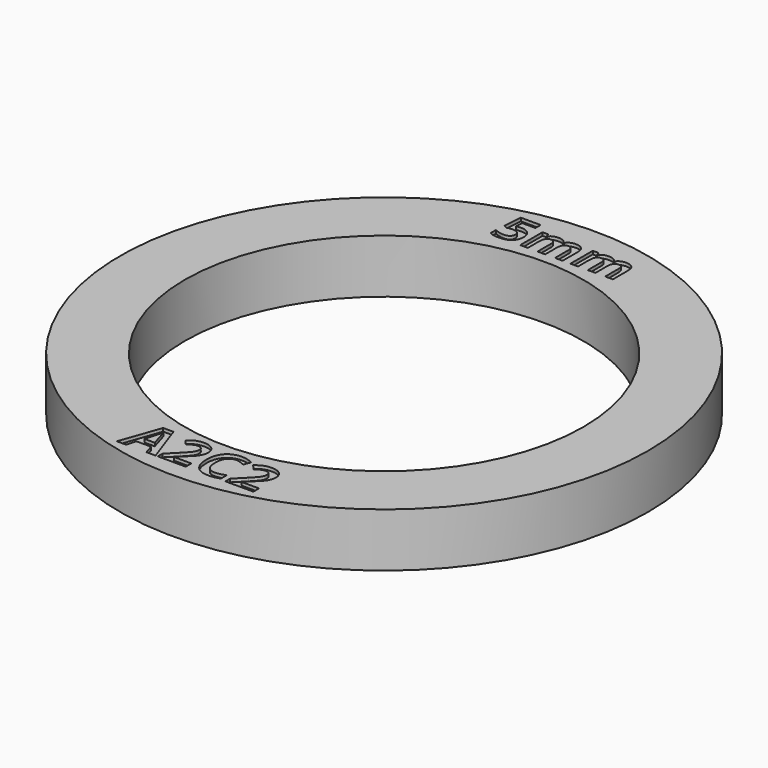
from build123d import *

# Parameters (mm, degrees)
F0_R           = 24.5
F0_R_2         = 18.5
F0_TEXT_SIZE   = 5.1974965673
F0_TEXT_SIZE_2 = 4.7515974277
F1_DEPTH       = 5
F2_DEPTH       = 0.3


# Not quite as in the source:
# - Text() gives the source's letters only with a copy of the font that has no kerning and outlines rounded to 1/6400 em; it was checked with that copy


with BuildPart() as f1:
    # F0 (on Top) → F1 (new body)
    with BuildSketch(Plane.XY):
        Circle(F0_R)
        Polygon((-2.9154707307, -22.8730905801), (-3.7633123583, -22.8730905801), (-4.0321203839, -21.9895161637), (-5.3850937091, -21.9895161637), (-5.6539017347, -22.8730905801), (-6.5017433622, -22.8730905801), (-5.1918118055, -19.1471352284), (-4.2302749405, -19.1471352284), align=None, mode=Mode.SUBTRACT)
        with BuildLine():
            Line((-0.1136952374, -22.2128460943), (-0.1136952374, -22.8730905801))
            Line((-0.1136952374, -22.8730905801), (-2.707570868, -22.8730905801))
            Line((-2.707570868, -22.8730905801), (-2.707570868, -22.3273534405))
            Line((-2.707570868, -22.3273534405), (-1.7760820301, -21.3861192965))
            add(Edge.make_bspline(
                [(-1.7760820301, -21.3861192965), (-1.3619065224, -20.9621984828), (-1.2352175436, -20.7985585518)],
                knots=[0, 0, 0, 1, 1, 1], degree=2))
            add(Edge.make_bspline(
                [(-1.2352175436, -20.7985585518), (-1.1085285648, -20.6349186208), (-1.0524930549, -20.4952359005)],
                knots=[0, 0, 0, 1, 1, 1], degree=2))
            add(Edge.make_bspline(
                [(-1.0524930549, -20.4952359005), (-0.996457545, -20.3555531803), (-0.996457545, -20.206125154)],
                knots=[0, 0, 0, 1, 1, 1], degree=2))
            add(Edge.make_bspline(
                [(-0.996457545, -20.206125154), (-0.996457545, -19.9827952234), (-1.1198980885, -19.8735665846)],
                knots=[0, 0, 0, 1, 1, 1], degree=2))
            add(Edge.make_bspline(
                [(-1.1198980885, -19.8735665846), (-1.243338632, -19.7643379458), (-1.4488021681, -19.7643379458)],
                knots=[0, 0, 0, 1, 1, 1], degree=2))
            add(Edge.make_bspline(
                [(-1.4488021681, -19.7643379458), (-1.6640110104, -19.7643379458), (-1.86703822, -19.8634152241)],
                knots=[0, 0, 0, 1, 1, 1], degree=2))
            add(Edge.make_bspline(
                [(-1.86703822, -19.8634152241), (-2.0700654297, -19.9624925024), (-2.2909590338, -20.1452169911)],
                knots=[0, 0, 0, 1, 1, 1], degree=2))
            Line((-2.2909590338, -20.1452169911), (-2.7173161741, -19.6400852935))
            add(Edge.make_bspline(
                [(-2.7173161741, -19.6400852935), (-2.4436354955, -19.4061979479), (-2.2633473333, -19.3099630505)],
                knots=[0, 0, 0, 1, 1, 1], degree=2))
            add(Edge.make_bspline(
                [(-2.2633473333, -19.3099630505), (-2.0830591711, -19.2137281532), (-1.869880601, -19.1617531875)],
                knots=[0, 0, 0, 1, 1, 1], degree=2))
            add(Edge.make_bspline(
                [(-1.869880601, -19.1617531875), (-1.6567020308, -19.1097782218), (-1.3927666583, -19.1097782218)],
                knots=[0, 0, 0, 1, 1, 1], degree=2))
            add(Edge.make_bspline(
                [(-1.3927666583, -19.1097782218), (-1.0451840753, -19.1097782218), (-0.7788123763, -19.2364672006)],
                knots=[0, 0, 0, 1, 1, 1], degree=2))
            add(Edge.make_bspline(
                [(-0.7788123763, -19.2364672006), (-0.5124406772, -19.3631561795), (-0.365042923, -19.5917648176)],
                knots=[0, 0, 0, 1, 1, 1], degree=2))
            add(Edge.make_bspline(
                [(-0.365042923, -19.5917648176), (-0.2176451688, -19.8203734556), (-0.2176451688, -20.1143568552)],
                knots=[0, 0, 0, 1, 1, 1], degree=2))
            add(Edge.make_bspline(
                [(-0.2176451688, -20.1143568552), (-0.2176451688, -20.3709832482), (-0.3077892498, -20.5955313421)],
                knots=[0, 0, 0, 1, 1, 1], degree=2))
            add(Edge.make_bspline(
                [(-0.3077892498, -20.5955313421), (-0.3979333309, -20.820079436), (-0.5871546903, -21.0559970536)],
                knots=[0, 0, 0, 1, 1, 1], degree=2))
            add(Edge.make_bspline(
                [(-0.5871546903, -21.0559970536), (-0.7763760497, -21.2919146713), (-1.253083938, -21.7288292265)],
                knots=[0, 0, 0, 1, 1, 1], degree=2))
            Line((-1.253083938, -21.7288292265), (-1.7306039352, -22.1779254142))
            Line((-1.7306039352, -22.1779254142), (-1.7306039352, -22.2128460943))
            Line((-1.7306039352, -22.2128460943), (-0.1136952374, -22.2128460943))
        make_face(mode=Mode.SUBTRACT)
        Circle(F0_R_2, mode=Mode.SUBTRACT)
        with BuildLine():
            add(Edge.make_bspline(
                [(2.5077920937, -19.8378337957), (2.2974559045, -19.7643379458), (2.0944286949, -19.7643379458)],
                knots=[0, 0, 0, 1, 1, 1], degree=2))
            add(Edge.make_bspline(
                [(2.0944286949, -19.7643379458), (1.6502051601, -19.7643379458), (1.4065725085, -20.0981146785)],
                knots=[0, 0, 0, 1, 1, 1], degree=2))
            add(Edge.make_bspline(
                [(1.4065725085, -20.0981146785), (1.1629398569, -20.4318914111), (1.1629398569, -21.0279792987)],
                knots=[0, 0, 0, 1, 1, 1], degree=2))
            add(Edge.make_bspline(
                [(1.1629398569, -21.0279792987), (1.1629398569, -22.2688816042), (2.0944286949, -22.2688816042)],
                knots=[0, 0, 0, 1, 1, 1], degree=2))
            add(Edge.make_bspline(
                [(2.0944286949, -22.2688816042), (2.4850530463, -22.2688816042), (3.0405354919, -22.0739754829)],
                knots=[0, 0, 0, 1, 1, 1], degree=2))
            Line((3.0405354919, -22.0739754829), (3.0405354919, -22.7334078599))
            add(Edge.make_bspline(
                [(3.0405354919, -22.7334078599), (2.5841303246, -22.9242534369), (2.0205267906, -22.9242534369)],
                knots=[0, 0, 0, 1, 1, 1], degree=2))
            add(Edge.make_bspline(
                [(2.0205267906, -22.9242534369), (1.2108542784, -22.9242534369), (0.7820608116, -22.4329275896)],
                knots=[0, 0, 0, 1, 1, 1], degree=2))
            add(Edge.make_bspline(
                [(0.7820608116, -22.4329275896), (0.3532673448, -21.9416017422), (0.3532673448, -21.0231066457)],
                knots=[0, 0, 0, 1, 1, 1], degree=2))
            add(Edge.make_bspline(
                [(0.3532673448, -21.0231066457), (0.3532673448, -20.4440730437), (0.5640095884, -20.0087827062)],
                knots=[0, 0, 0, 1, 1, 1], degree=2))
            add(Edge.make_bspline(
                [(0.5640095884, -20.0087827062), (0.7747518321, -19.5734923687), (1.1694367277, -19.3416352953)],
                knots=[0, 0, 0, 1, 1, 1], degree=2))
            add(Edge.make_bspline(
                [(1.1694367277, -19.3416352953), (1.5641216232, -19.1097782218), (2.0944286949, -19.1097782218)],
                knots=[0, 0, 0, 1, 1, 1], degree=2))
            add(Edge.make_bspline(
                [(2.0944286949, -19.1097782218), (2.6344810726, -19.1097782218), (3.1802182121, -19.370465159)],
                knots=[0, 0, 0, 1, 1, 1], degree=2))
            Line((3.1802182121, -19.370465159), (2.9268402545, -20.0104069239))
            add(Edge.make_bspline(
                [(2.9268402545, -20.0104069239), (2.7181282829, -19.9113296456), (2.5077920937, -19.8378337957)],
                knots=[0, 0, 0, 1, 1, 1], degree=2))
        make_face(mode=Mode.SUBTRACT)
        with BuildLine():
            Line((6.1647181942, -22.2128460943), (6.1647181942, -22.8730905801))
            Line((6.1647181942, -22.8730905801), (3.5708425635, -22.8730905801))
            Line((3.5708425635, -22.8730905801), (3.5708425635, -22.3273534405))
            Line((3.5708425635, -22.3273534405), (4.5023314015, -21.3861192965))
            add(Edge.make_bspline(
                [(4.5023314015, -21.3861192965), (4.9165069092, -20.9621984828), (5.043195888, -20.7985585518)],
                knots=[0, 0, 0, 1, 1, 1], degree=2))
            add(Edge.make_bspline(
                [(5.043195888, -20.7985585518), (5.1698848668, -20.6349186208), (5.2259203767, -20.4952359005)],
                knots=[0, 0, 0, 1, 1, 1], degree=2))
            add(Edge.make_bspline(
                [(5.2259203767, -20.4952359005), (5.2819558866, -20.3555531803), (5.2819558866, -20.206125154)],
                knots=[0, 0, 0, 1, 1, 1], degree=2))
            add(Edge.make_bspline(
                [(5.2819558866, -20.206125154), (5.2819558866, -19.9827952234), (5.1585153431, -19.8735665846)],
                knots=[0, 0, 0, 1, 1, 1], degree=2))
            add(Edge.make_bspline(
                [(5.1585153431, -19.8735665846), (5.0350747996, -19.7643379458), (4.8296112634, -19.7643379458)],
                knots=[0, 0, 0, 1, 1, 1], degree=2))
            add(Edge.make_bspline(
                [(4.8296112634, -19.7643379458), (4.6144024212, -19.7643379458), (4.4113752115, -19.8634152241)],
                knots=[0, 0, 0, 1, 1, 1], degree=2))
            add(Edge.make_bspline(
                [(4.4113752115, -19.8634152241), (4.2083480019, -19.9624925024), (3.9874543978, -20.1452169911)],
                knots=[0, 0, 0, 1, 1, 1], degree=2))
            Line((3.9874543978, -20.1452169911), (3.5610972575, -19.6400852935))
            add(Edge.make_bspline(
                [(3.5610972575, -19.6400852935), (3.8347779361, -19.4061979479), (4.0150660983, -19.3099630505)],
                knots=[0, 0, 0, 1, 1, 1], degree=2))
            add(Edge.make_bspline(
                [(4.0150660983, -19.3099630505), (4.1953542604, -19.2137281532), (4.4085328306, -19.1617531875)],
                knots=[0, 0, 0, 1, 1, 1], degree=2))
            add(Edge.make_bspline(
                [(4.4085328306, -19.1617531875), (4.6217114007, -19.1097782218), (4.8856467733, -19.1097782218)],
                knots=[0, 0, 0, 1, 1, 1], degree=2))
            add(Edge.make_bspline(
                [(4.8856467733, -19.1097782218), (5.2332293562, -19.1097782218), (5.4996010553, -19.2364672006)],
                knots=[0, 0, 0, 1, 1, 1], degree=2))
            add(Edge.make_bspline(
                [(5.4996010553, -19.2364672006), (5.7659727544, -19.3631561795), (5.9133705086, -19.5917648176)],
                knots=[0, 0, 0, 1, 1, 1], degree=2))
            add(Edge.make_bspline(
                [(5.9133705086, -19.5917648176), (6.0607682628, -19.8203734556), (6.0607682628, -20.1143568552)],
                knots=[0, 0, 0, 1, 1, 1], degree=2))
            add(Edge.make_bspline(
                [(6.0607682628, -20.1143568552), (6.0607682628, -20.3709832482), (5.9706241817, -20.5955313421)],
                knots=[0, 0, 0, 1, 1, 1], degree=2))
            add(Edge.make_bspline(
                [(5.9706241817, -20.5955313421), (5.8804801006, -20.820079436), (5.6912587412, -21.0559970536)],
                knots=[0, 0, 0, 1, 1, 1], degree=2))
            add(Edge.make_bspline(
                [(5.6912587412, -21.0559970536), (5.5020373818, -21.2919146713), (5.0253294935, -21.7288292265)],
                knots=[0, 0, 0, 1, 1, 1], degree=2))
            Line((5.0253294935, -21.7288292265), (4.5478094964, -22.1779254142))
            Line((4.5478094964, -22.1779254142), (4.5478094964, -22.2128460943))
            Line((4.5478094964, -22.2128460943), (6.1647181942, -22.2128460943))
        make_face(mode=Mode.SUBTRACT)
        with BuildLine():
            add(Edge.make_bspline(
                [(-4.9238428344, 21.5662038617), (-4.7820373487, 21.598871094), (-4.5734125241, 21.598871094)],
                knots=[0, 0, 0, 1, 1, 1], degree=2))
            add(Edge.make_bspline(
                [(-4.5734125241, 21.598871094), (-4.0819191652, 21.598871094), (-3.7905126042, 21.3226844935)],
                knots=[0, 0, 0, 1, 1, 1], degree=2))
            add(Edge.make_bspline(
                [(-3.7905126042, 21.3226844935), (-3.4991060432, 21.046497893), (-3.4991060432, 20.5661410906)],
                knots=[0, 0, 0, 1, 1, 1], degree=2))
            add(Edge.make_bspline(
                [(-3.4991060432, 20.5661410906), (-3.4991060432, 19.9981767105), (-3.8495363535, 19.691550189)],
                knots=[0, 0, 0, 1, 1, 1], degree=2))
            add(Edge.make_bspline(
                [(-3.8495363535, 19.691550189), (-4.1999666638, 19.3849236675), (-4.8518264359, 19.3849236675)],
                knots=[0, 0, 0, 1, 1, 1], degree=2))
            add(Edge.make_bspline(
                [(-4.8518264359, 19.3849236675), (-5.4183059417, 19.3849236675), (-5.7657665036, 19.5683056308)],
                knots=[0, 0, 0, 1, 1, 1], degree=2))
            Line((-5.7657665036, 19.5683056308), (-5.7657665036, 20.1882406076))
            add(Edge.make_bspline(
                [(-5.7657665036, 20.1882406076), (-5.5831269775, 20.0909813478), (-5.3392363908, 20.0293590687)],
                knots=[0, 0, 0, 1, 1, 1], degree=2))
            add(Edge.make_bspline(
                [(-5.3392363908, 20.0293590687), (-5.0953458041, 19.9677367895), (-4.8778117343, 19.9677367895)],
                knots=[0, 0, 0, 1, 1, 1], degree=2))
            add(Edge.make_bspline(
                [(-4.8778117343, 19.9677367895), (-4.2207549025, 19.9677367895), (-4.2207549025, 20.5060036856)],
                knots=[0, 0, 0, 1, 1, 1], degree=2))
            add(Edge.make_bspline(
                [(-4.2207549025, 20.5060036856), (-4.2207549025, 21.0190277204), (-4.9008272844, 21.0190277204)],
                knots=[0, 0, 0, 1, 1, 1], degree=2))
            add(Edge.make_bspline(
                [(-4.9008272844, 21.0190277204), (-5.0233294056, 21.0190277204), (-5.1718168252, 20.9945272962)],
                knots=[0, 0, 0, 1, 1, 1], degree=2))
            add(Edge.make_bspline(
                [(-5.1718168252, 20.9945272962), (-5.3203042448, 20.9700268719), (-5.413108882, 20.9418142622)],
                knots=[0, 0, 0, 1, 1, 1], degree=2))
            Line((-5.413108882, 20.9418142622), (-5.6989471648, 21.0954987415))
            Line((-5.6989471648, 21.0954987415), (-5.5712479839, 22.8238923058))
            Line((-5.5712479839, 22.8238923058), (-3.7314888549, 22.8238923058))
            Line((-3.7314888549, 22.8238923058), (-3.7314888549, 22.2158363225))
            Line((-3.7314888549, 22.2158363225), (-4.9424037619, 22.2158363225))
            Line((-4.9424037619, 22.2158363225), (-5.0047684781, 21.5498702455))
            Line((-5.0047684781, 21.5498702455), (-4.9238428344, 21.5662038617))
        make_face(mode=Mode.SUBTRACT)
        with BuildLine():
            Line((-0.5924648043, 20.7331894376), (-0.5924648043, 19.4316972047))
            Line((-0.5924648043, 19.4316972047), (-1.3000073587, 19.4316972047))
            Line((-1.3000073587, 19.4316972047), (-1.3000073587, 20.9470113219))
            add(Edge.make_bspline(
                [(-1.3000073587, 20.9470113219), (-1.3000073587, 21.2276525449), (-1.3939256516, 21.3679731565)],
                knots=[0, 0, 0, 1, 1, 1], degree=2))
            add(Edge.make_bspline(
                [(-1.3939256516, 21.3679731565), (-1.4878439445, 21.508293768), (-1.6897868352, 21.508293768)],
                knots=[0, 0, 0, 1, 1, 1], degree=2))
            add(Edge.make_bspline(
                [(-1.6897868352, 21.508293768), (-1.9615188131, 21.508293768), (-2.0843921528, 21.3085781886)],
                knots=[0, 0, 0, 1, 1, 1], degree=2))
            add(Edge.make_bspline(
                [(-2.0843921528, 21.3085781886), (-2.2072654926, 21.1088626093), (-2.2072654926, 20.6522637939)],
                knots=[0, 0, 0, 1, 1, 1], degree=2))
            Line((-2.2072654926, 20.6522637939), (-2.2072654926, 19.4316972047))
            Line((-2.2072654926, 19.4316972047), (-2.914808047, 19.4316972047))
            Line((-2.914808047, 19.4316972047), (-2.914808047, 22.0257724254))
            Line((-2.914808047, 22.0257724254), (-2.3743138396, 22.0257724254))
            Line((-2.3743138396, 22.0257724254), (-2.2792818911, 21.6939030425))
            Line((-2.2792818911, 21.6939030425), (-2.2399327249, 21.6939030425))
            add(Edge.make_bspline(
                [(-2.2399327249, 21.6939030425), (-2.1352490941, 21.8728303832), (-1.9381320445, 21.97343061)],
                knots=[0, 0, 0, 1, 1, 1], degree=2))
            add(Edge.make_bspline(
                [(-1.9381320445, 21.97343061), (-1.741014995, 22.0740308367), (-1.4856166332, 22.0740308367)],
                knots=[0, 0, 0, 1, 1, 1], degree=2))
            add(Edge.make_bspline(
                [(-1.4856166332, 22.0740308367), (-0.9035459484, 22.0740308367), (-0.696405998, 21.6939030425)],
                knots=[0, 0, 0, 1, 1, 1], degree=2))
            Line((-0.696405998, 21.6939030425), (-0.6340412818, 21.6939030425))
            add(Edge.make_bspline(
                [(-0.6340412818, 21.6939030425), (-0.5293576509, 21.8750576945), (-0.3266723232, 21.9745442656)],
                knots=[0, 0, 0, 1, 1, 1], degree=2))
            add(Edge.make_bspline(
                [(-0.3266723232, 21.9745442656), (-0.1239869954, 22.0740308367), (0.1314113664, 22.0740308367)],
                knots=[0, 0, 0, 1, 1, 1], degree=2))
            add(Edge.make_bspline(
                [(0.1314113664, 22.0740308367), (0.5724190026, 22.0740308367), (0.798491099, 21.8479587404)],
                knots=[0, 0, 0, 1, 1, 1], degree=2))
            add(Edge.make_bspline(
                [(0.798491099, 21.8479587404), (1.0245631953, 21.621886644), (1.0245631953, 21.1229689141)],
                knots=[0, 0, 0, 1, 1, 1], degree=2))
            Line((1.0245631953, 21.1229689141), (1.0245631953, 19.4316972047))
            Line((1.0245631953, 19.4316972047), (0.3147933296, 19.4316972047))
            Line((0.3147933296, 19.4316972047), (0.3147933296, 20.9470113219))
            add(Edge.make_bspline(
                [(0.3147933296, 20.9470113219), (0.3147933296, 21.2276525449), (0.2208750367, 21.3679731565)],
                knots=[0, 0, 0, 1, 1, 1], degree=2))
            add(Edge.make_bspline(
                [(0.2208750367, 21.3679731565), (0.1269567438, 21.508293768), (-0.0749861469, 21.508293768)],
                knots=[0, 0, 0, 1, 1, 1], degree=2))
            add(Edge.make_bspline(
                [(-0.0749861469, 21.508293768), (-0.3348391312, 21.508293768), (-0.4636519677, 21.3226844935)],
                knots=[0, 0, 0, 1, 1, 1], degree=2))
            add(Edge.make_bspline(
                [(-0.4636519677, 21.3226844935), (-0.5924648043, 21.137075219), (-0.5924648043, 20.7331894376)],
                knots=[0, 0, 0, 1, 1, 1], degree=2))
        make_face(mode=Mode.SUBTRACT)
        with BuildLine():
            Line((4.07300992, 20.7331894376), (4.07300992, 19.4316972047))
            Line((4.07300992, 19.4316972047), (3.3654673656, 19.4316972047))
            Line((3.3654673656, 19.4316972047), (3.3654673656, 20.9470113219))
            add(Edge.make_bspline(
                [(3.3654673656, 20.9470113219), (3.3654673656, 21.2276525449), (3.2715490727, 21.3679731565)],
                knots=[0, 0, 0, 1, 1, 1], degree=2))
            add(Edge.make_bspline(
                [(3.2715490727, 21.3679731565), (3.1776307797, 21.508293768), (2.9756878891, 21.508293768)],
                knots=[0, 0, 0, 1, 1, 1], degree=2))
            add(Edge.make_bspline(
                [(2.9756878891, 21.508293768), (2.7039559112, 21.508293768), (2.5810825714, 21.3085781886)],
                knots=[0, 0, 0, 1, 1, 1], degree=2))
            add(Edge.make_bspline(
                [(2.5810825714, 21.3085781886), (2.4582092317, 21.1088626093), (2.4582092317, 20.6522637939)],
                knots=[0, 0, 0, 1, 1, 1], degree=2))
            Line((2.4582092317, 20.6522637939), (2.4582092317, 19.4316972047))
            Line((2.4582092317, 19.4316972047), (1.7506666773, 19.4316972047))
            Line((1.7506666773, 19.4316972047), (1.7506666773, 22.0257724254))
            Line((1.7506666773, 22.0257724254), (2.2911608846, 22.0257724254))
            Line((2.2911608846, 22.0257724254), (2.3861928332, 21.6939030425))
            Line((2.3861928332, 21.6939030425), (2.4255419994, 21.6939030425))
            add(Edge.make_bspline(
                [(2.4255419994, 21.6939030425), (2.5302256302, 21.8728303832), (2.7273426798, 21.97343061)],
                knots=[0, 0, 0, 1, 1, 1], degree=2))
            add(Edge.make_bspline(
                [(2.7273426798, 21.97343061), (2.9244597293, 22.0740308367), (3.179858091, 22.0740308367)],
                knots=[0, 0, 0, 1, 1, 1], degree=2))
            add(Edge.make_bspline(
                [(3.179858091, 22.0740308367), (3.7619287759, 22.0740308367), (3.9690687263, 21.6939030425)],
                knots=[0, 0, 0, 1, 1, 1], degree=2))
            Line((3.9690687263, 21.6939030425), (4.0314334425, 21.6939030425))
            add(Edge.make_bspline(
                [(4.0314334425, 21.6939030425), (4.1361170734, 21.8750576945), (4.3388024011, 21.9745442656)],
                knots=[0, 0, 0, 1, 1, 1], degree=2))
            add(Edge.make_bspline(
                [(4.3388024011, 21.9745442656), (4.5414877289, 22.0740308367), (4.7968860906, 22.0740308367)],
                knots=[0, 0, 0, 1, 1, 1], degree=2))
            add(Edge.make_bspline(
                [(4.7968860906, 22.0740308367), (5.2378937269, 22.0740308367), (5.4639658233, 21.8479587404)],
                knots=[0, 0, 0, 1, 1, 1], degree=2))
            add(Edge.make_bspline(
                [(5.4639658233, 21.8479587404), (5.6900379196, 21.621886644), (5.6900379196, 21.1229689141)],
                knots=[0, 0, 0, 1, 1, 1], degree=2))
            Line((5.6900379196, 21.1229689141), (5.6900379196, 19.4316972047))
            Line((5.6900379196, 19.4316972047), (4.9802680539, 19.4316972047))
            Line((4.9802680539, 19.4316972047), (4.9802680539, 20.9470113219))
            add(Edge.make_bspline(
                [(4.9802680539, 20.9470113219), (4.9802680539, 21.2276525449), (4.886349761, 21.3679731565)],
                knots=[0, 0, 0, 1, 1, 1], degree=2))
            add(Edge.make_bspline(
                [(4.886349761, 21.3679731565), (4.7924314681, 21.508293768), (4.5904885774, 21.508293768)],
                knots=[0, 0, 0, 1, 1, 1], degree=2))
            add(Edge.make_bspline(
                [(4.5904885774, 21.508293768), (4.3306355931, 21.508293768), (4.2018227565, 21.3226844935)],
                knots=[0, 0, 0, 1, 1, 1], degree=2))
            add(Edge.make_bspline(
                [(4.2018227565, 21.3226844935), (4.07300992, 21.137075219), (4.07300992, 20.7331894376)],
                knots=[0, 0, 0, 1, 1, 1], degree=2))
        make_face(mode=Mode.SUBTRACT)
        with BuildLine():
            Line((-5.1869391524, -21.3300837867), (-4.2205296344, -21.3300837867))
            add(Edge.make_bspline(
                [(-4.2205296344, -21.3300837867), (-4.5932875914, -20.1297869232), (-4.640389904, -19.9722378085)],
                knots=[0, 0, 0, 1, 1, 1], degree=2))
            add(Edge.make_bspline(
                [(-4.640389904, -19.9722378085), (-4.6874922167, -19.8146886938), (-4.7077949376, -19.7237325038)],
                knots=[0, 0, 0, 1, 1, 1], degree=2))
            add(Edge.make_bspline(
                [(-4.7077949376, -19.7237325038), (-4.791442148, -20.0485760393), (-5.1869391524, -21.3300837867)],
                knots=[0, 0, 0, 1, 1, 1], degree=2))
        make_face()
        with Locations((-6.5017433622, -22.8730905801)):
            Text('A2C2', F0_TEXT_SIZE, font='Open Sans', font_style=FontStyle.BOLD, text_align=(TextAlign.LEFT, TextAlign.BOTTOM))
        with Locations((-5.9981493153, 19.4316972047)):
            Text('5mm', F0_TEXT_SIZE_2, font='Open Sans', font_style=FontStyle.BOLD, text_align=(TextAlign.LEFT, TextAlign.BOTTOM))
    extrude(amount=-F1_DEPTH)

    # F0 (on Top) → F2 (cut)
    with BuildSketch(Plane.XY):
        with Locations((-6.5017433622, -22.8730905801)):
            Text('A2C2', F0_TEXT_SIZE, font='Open Sans', font_style=FontStyle.BOLD, text_align=(TextAlign.LEFT, TextAlign.BOTTOM))
        with Locations((-5.9981493153, 19.4316972047)):
            Text('5mm', F0_TEXT_SIZE_2, font='Open Sans', font_style=FontStyle.BOLD, text_align=(TextAlign.LEFT, TextAlign.BOTTOM))
    extrude(amount=-F2_DEPTH, mode=Mode.SUBTRACT)


solid = f1.part
